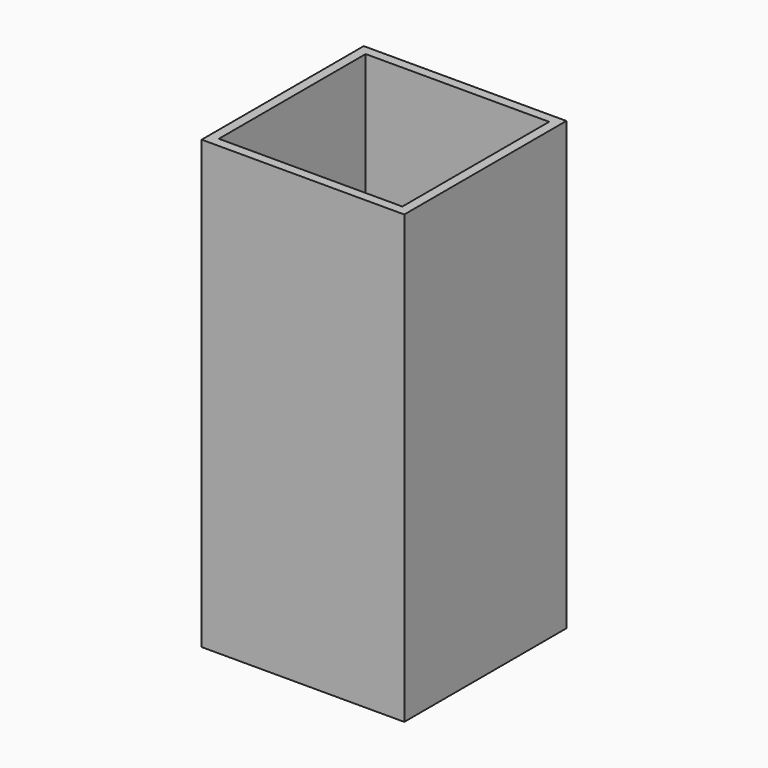
from build123d import *

# Parameters (mm, degrees)
F0_W     = 63.5
F0_H     = 63.5
F0_W_2   = 57.5
F0_H_2   = 57.5
F1_DEPTH = 140
F2_R     = 10
F3_DEPTH = 3


# Not quite as in the source:
# - a feature names something its author has since deleted; it is built from what else it names


with BuildPart() as f1:
    # F0 (on Top) → F1 (new body)
    with BuildSketch(Plane.XY):
        with Locations((2.4368530139, 1.7202482249)):
            Rectangle(F0_W, F0_H)
        with Locations((2.4368530139, 1.7202482249)):
            Rectangle(F0_W_2, F0_H_2, mode=Mode.SUBTRACT)
    extrude(amount=F1_DEPTH)

    # F2 (on face) → F3 (cut)
    with BuildSketch(Plane(origin=(-29.3131469861, 0, 0), x_dir=(0, -1, 0), z_dir=(-1, 0, 0))):
        with Locations((-1.7202482249, 20)):
            Circle(F2_R)
    extrude(amount=-F3_DEPTH, mode=Mode.SUBTRACT)


solid = f1.part
